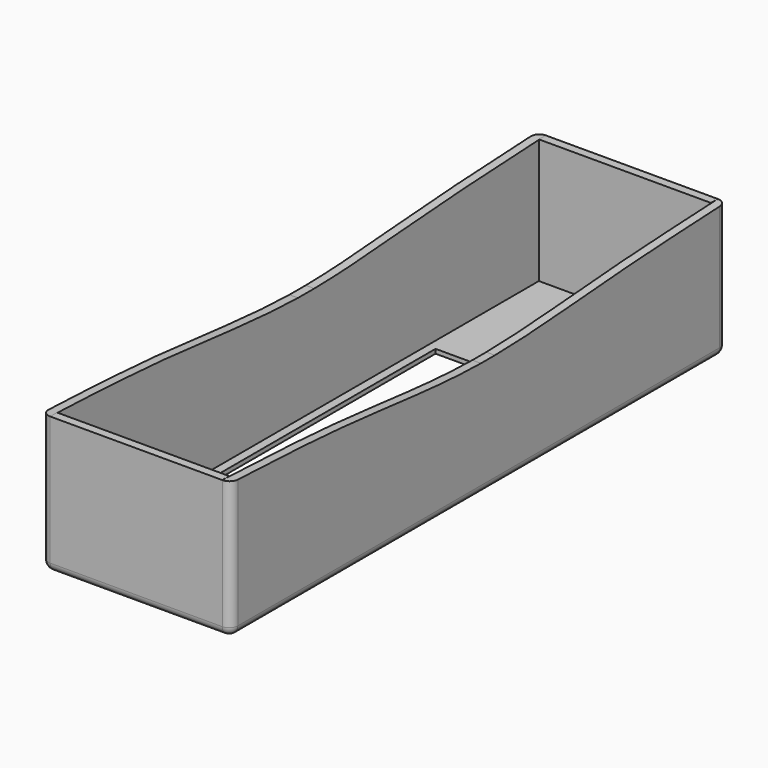
from build123d import *

# Parameters (mm, degrees)
F0_W      = 44
F0_H      = 144
F0_W_2    = 40
F0_H_2    = 140
F1_DEPTH  = 2
F2_DEPTH  = 25
F5_DEPTH  = 2
F6_DEPTH  = 2
F7_DEPTH  = 5
F8_DEPTH  = 4
F10_DEPTH = 32.0010001
F9_W      = 36
F9_H      = 2
F9_W_2    = 2
F9_H_2    = 73
F11_DEPTH = 1
F12_R     = 1.99999


# Not quite as in the source:
# - a fillet or chamfer is up to 0.001 mm smaller than in the source, because OpenCascade refuses the exact size


with BuildPart() as f1:
    # F0 (on Top) → F1 (new body)
    with BuildSketch(Plane.XY):
        Rectangle(F0_W, F0_H)
        Rectangle(F0_W_2, F0_H_2, mode=Mode.SUBTRACT)
        Rectangle(F0_W_2, F0_H_2)
    extrude(amount=-F1_DEPTH)

    # F0 (on Top) → F2 (join)
    with BuildSketch(Plane.XY):
        Rectangle(F0_W, F0_H)
        Rectangle(F0_W_2, F0_H_2, mode=Mode.SUBTRACT)
    extrude(amount=F2_DEPTH)

    # F3 (on face) → F5 (join)
    with BuildSketch(Plane.YZ.offset(22)):
        with BuildLine():
            add(Edge.make_bspline(
                [(4.7271151019, 25), (15.348527654, 25.1268953042), (37.9929862917, 27.4159301893), (60.2495129104, 28.4605212291), (72, 29)],
                knots=[0.5326300299, 0.5326300299, 0.5326300299, 0.5326300299, 0.7517880542, 1, 1, 1, 1], degree=3))
            Line((4.7271151019, 25), (72, 25))
            Line((72, 25), (72, 29))
        make_face()
        with BuildLine():
            Line((-72, 30), (-72, 25))
            Line((-72, 25), (0.6763282883, 25))
            add(Edge.make_bspline(
                [(-72, 30), (-60.2445668251, 29.5430569498), (-36.4192696174, 28.5876982607), (-11.9822251211, 25.1864507884), (0.4508819142, 25.0028330974), (0.6763282883, 25)],
                knots=[0, 0, 0, 0, 0.2482119458, 0.5001170824, 0.504769099, 0.504769099, 0.504769099, 0.504769099], degree=3))
        make_face()
    extrude(amount=-F5_DEPTH)

    # F4 (on face) → F6 (join)
    with BuildSketch(Plane(origin=(-22, 0, 0), x_dir=(0, -1, 0), z_dir=(-1, 0, 0))):
        with BuildLine():
            Line((-72, 29), (-72, 25))
            Line((-72, 25), (-4.7271151019, 25))
            add(Edge.make_bspline(
                [(-72, 29), (-60.2495129104, 28.4605212291), (-37.9929862917, 27.4159301893), (-15.348527654, 25.1268953042), (-4.7271151019, 25)],
                knots=[0, 0, 0, 0, 0.2482119458, 0.4673699701, 0.4673699701, 0.4673699701, 0.4673699701], degree=3))
        make_face()
        with BuildLine():
            Line((0, 25), (72, 25))
            Line((72, 25), (72, 30))
            add(Edge.make_bspline(
                [(0, 25.01), (12.2074400514, 25.2177971205), (36.4192696174, 28.5876982607), (60.2445668251, 29.5430569498), (72, 30)],
                knots=[0.4998829176, 0.4998829176, 0.4998829176, 0.4998829176, 0.7517880542, 1, 1, 1, 1], degree=3))
            Line((0, 25.01), (0, 25))
        make_face()
    extrude(amount=-F6_DEPTH)

    # F7 (add): a face of the model
    f7_faces = [f1.faces().sort_by_distance(p)[0] for p in [
        (0, -71, 25),
    ]]
    extrude(f7_faces, amount=F7_DEPTH)

    # F8 (add): a face of the model
    f8_faces = [f1.faces().sort_by_distance(p)[0] for p in [
        (0, 71, 25),
    ]]
    extrude(f8_faces, amount=F8_DEPTH)

    # F9 (on face) → F10 (cut, through all)
    with BuildSketch(Plane(origin=(0, 0, -2), x_dir=(1, 0, 0), z_dir=(0, 0, -1))):
        Polygon((20, 35.5240486562), (20, 60.5240486562), (-20, 60.5240486562), (-20, 35.5240486562), (-18, 35.5240486562), (-18, -37.4759513438), (18, -37.4759513438), (18, 35.5240486562), align=None)
    extrude(amount=-F10_DEPTH, mode=Mode.SUBTRACT)

    # F9 (on face) → F11 (cut)
    with BuildSketch(Plane(origin=(0, 0, -2), x_dir=(1, 0, 0), z_dir=(0, 0, -1))):
        with Locations((0, -38.4759513438)):
            Rectangle(F9_W, F9_H)
        with Locations((-19, -38.4759513438)):
            Rectangle(F9_W_2, F9_H)
        with Locations((-19, -0.9759513438)):
            Rectangle(F9_W_2, F9_H_2)
        with Locations((19, -38.4759513438)):
            Rectangle(F9_W_2, F9_H)
        with Locations((19, -0.9759513438)):
            Rectangle(F9_W_2, F9_H_2)
    extrude(amount=-F11_DEPTH, mode=Mode.SUBTRACT)

    # F12 (radius 2 in the source; OpenCascade refuses exactly that, so slightly less here)
    f12_edges = [f1.edges().sort_by_distance(p)[0] for p in [
        (0, -72, -2),
        (-22, 0, -2),
        (22, 0, -2),
        (-22, -72, 14),
        (22, -72, 14),
        (0, 72, -2),
        (-22, 72, 13.5),
        (22, 72, 13.5),
    ]]
    fillet(f12_edges, radius=F12_R)


solid = f1.part
